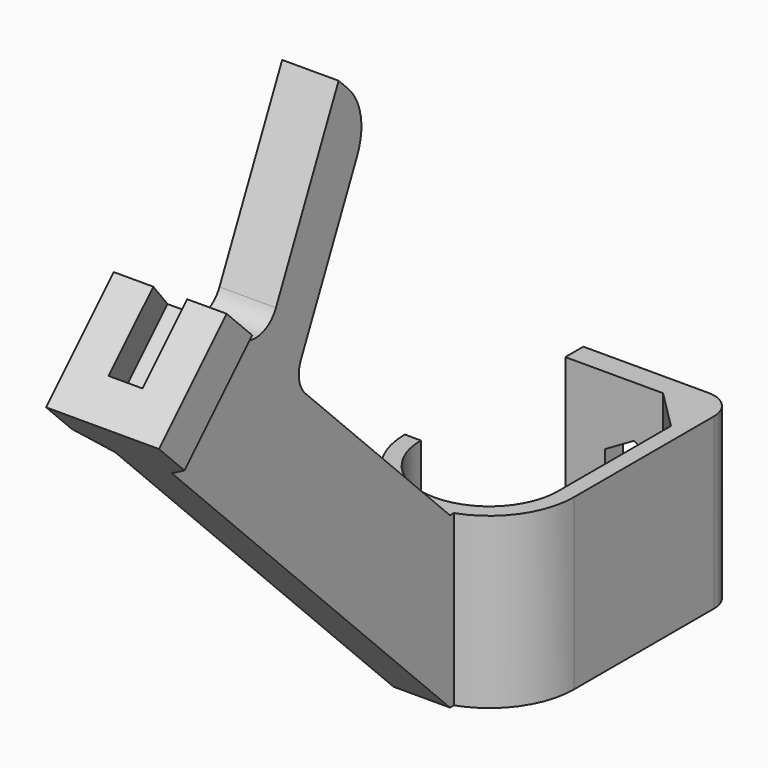
from build123d import *

# Parameters (mm, degrees)
F1_DEPTH  = 38.1
F2_W      = 3.6068
F2_H      = 38.1
F3_DEPTH  = 6.35
F5_DEPTH  = 12.7
F6_R      = 6.35
F7_R      = 12.7
F8_W      = 6.35
F8_H      = 10.16
F9_DEPTH  = 26.9407683632
F11_DEPTH = 17.78
F13_DEPTH = 25.4


# Not quite as in the source:
# - a feature names something its author has since deleted; it is built from what else it names


with BuildPart() as f1:
    # F0 (on Top) → F1 (new body)
    with BuildSketch(Plane.XY):
        with BuildLine():
            ThreePointArc((15.4432, 0), (0, -15.4432), (-15.4432, 0))
            Line((-15.4432, 0), (-19.05, 0))
            ThreePointArc((-19.05, 0), (0, -19.05), (19.05, 0))
            Line((19.05, 0), (19.05, 39.37))
            ThreePointArc((19.05, 39.37), (17.1901280605, 43.8601280605), (12.7, 45.72))
            Line((12.7, 45.72), (-15.4432, 45.72))
            Line((-15.4432, 45.72), (-15.4432, 40.64))
            Line((-15.4432, 40.64), (6.5532, 40.64))
            Line((6.5532, 40.64), (9.0932, 40.64))
            Line((9.0932, 40.64), (15.4432, 40.64))
            Line((15.4432, 40.64), (15.4432, 34.29))
            Line((15.4432, 34.29), (15.4432, 31.75))
            Line((15.4432, 31.75), (15.4432, 0))
        make_face()
        with BuildLine():
            Line((6.5532, 40.64), (15.4432, 31.75))
            Line((15.4432, 31.75), (15.4432, 34.29))
            ThreePointArc((15.4432, 34.29), (13.5833280605, 38.7801280605), (9.0932, 40.64))
            Line((9.0932, 40.64), (6.5532, 40.64))
        make_face()
        with BuildLine():
            ThreePointArc((9.0932, 40.64), (13.5833280605, 38.7801280605), (15.4432, 34.29))
            Line((15.4432, 34.29), (15.4432, 40.64))
            Line((15.4432, 40.64), (9.0932, 40.64))
        make_face()
    extrude(amount=F1_DEPTH)

    # F2 (on Right) → F3 (join, symmetric)
    with BuildSketch(Plane.YZ):
        Polygon((-108.8525612107, 89.8025612107), (-19.05, 0), (-19.05, 38.1), (-89.8025612107, 108.8525612107), align=None)
        with Locations((-17.2466, 19.05)):
            Rectangle(F2_W, F2_H)
    extrude(amount=F3_DEPTH, both=True)

    # F4 (on face) → F5 (join, through all)
    with BuildSketch(Plane.YZ.offset(6.35)):
        Polygon((-50.3730412721, 136.93248455), (-71.8420489686, 90.8920489686), (-62.8617928475, 81.9117928475), (-41.3927851511, 127.9522284289), align=None)
    extrude(amount=-F5_DEPTH)

    # F6
    f6_edges = [f1.edges().sort_by_distance(p)[0] for p in [
        (0, -71.842049, 90.892049),
        (0, -62.861793, 81.911793),
    ]]
    fillet(f6_edges, radius=F6_R)

    # F7
    f7_edges = [f1.edges().sort_by_distance(p)[0] for p in [
        (0, -41.392785, 127.952228),
    ]]
    fillet(f7_edges, radius=F7_R)

    # F8 (on face) → F9 (join, through all)
    with BuildSketch(Plane(origin=(0, 9.525, 9.525), x_dir=(1, 0, 0), z_dir=(0, 0.7071067812, 0.7071067812))):
        with Locations((-9.525, -135.3903841816)):
            Rectangle(F8_W, F8_H)
        with Locations((9.525, -135.3903841816)):
            Rectangle(F8_W, F8_H)
        Polygon((-12.7, -130.3103841816), (-6.35, -130.3103841816), (-6.35, -124.1391240244), align=None)
        Polygon((6.35, -124.1391240244), (6.35, -130.3103841816), (12.7, -130.3103841816), align=None)
    extrude(amount=-F9_DEPTH)

    # F10 (on face) → F11 (cut)
    with BuildSketch(Plane(origin=(0, 9.525, 9.525), x_dir=(1, 0, 0), z_dir=(0, 0.7071067812, 0.7071067812))):
        Polygon((-6.35, -130.3103841816), (-3.81, -140.4703841816), (0, -140.4703841816), (0, -130.3103841816), align=None)
        Polygon((0, -130.3103841816), (0, -140.4703841816), (3.81, -140.4703841816), (6.35, -130.3103841816), align=None)
    extrude(amount=-F11_DEPTH, mode=Mode.SUBTRACT)

    # F12 (on face) → F13 (cut)
    with BuildSketch(Plane(origin=(0, 45.72, 0), x_dir=(-1, 0, 0), z_dir=(0, 1, 0))):
        with BuildLine():
            Line((-6.477, 15.3105023065), (-3.2384999613, 13.4407534373))
            ThreePointArc((-3.2384999613, 13.4407534373), (-5.6092465291, 15.8114999806), (-6.477, 19.05))
            Line((-6.477, 19.05), (-6.477, 15.3105023065))
        make_face()
        with BuildLine():
            Line((-3.2384999613, 13.4407534373), (0, 11.5710046129))
            Line((0, 11.5710046129), (0, 12.573))
            ThreePointArc((0, 12.573), (-1.6763709335, 12.7936984173), (-3.2384999613, 13.4407534373))
        make_face()
        with BuildLine():
            Line((0, 12.573), (0, 11.5710046129))
            Line((0, 11.5710046129), (3.2384995854, 13.4407532203))
            ThreePointArc((3.2384995854, 13.4407532203), (1.6763707239, 12.7936983612), (0, 12.573))
        make_face()
        with BuildLine():
            ThreePointArc((6.477, 19.05), (5.6092464206, 15.8114997927), (3.2384995854, 13.4407532203))
            Line((3.2384995854, 13.4407532203), (6.477, 15.3105023065))
            Line((6.477, 15.3105023065), (6.477, 19.05))
        make_face()
        with BuildLine():
            ThreePointArc((3.2384999681, 24.6592465587), (5.6092465311, 22.288500016), (6.477, 19.05))
            Line((6.477, 19.05), (6.477, 22.7894976935))
            Line((6.477, 22.7894976935), (3.2384999681, 24.6592465587))
        make_face()
        with BuildLine():
            Line((-6.477, 22.7894976935), (-6.477, 19.05))
            ThreePointArc((-6.477, 19.05), (-5.6092466761, 22.2884997648), (-3.2385004704, 24.6592462687))
            Line((-3.2385004704, 24.6592462687), (-6.477, 22.7894976935))
        make_face()
        with BuildLine():
            ThreePointArc((-3.2385004704, 24.6592462687), (-1.6763712174, 25.3063015066), (0, 25.527))
            Line((0, 25.527), (0, 26.5289953871))
            Line((0, 26.5289953871), (-3.2385004704, 24.6592462687))
        make_face()
        with BuildLine():
            ThreePointArc((0, 25.527), (1.6763709373, 25.3063015816), (3.2384999681, 24.6592465587))
            Line((3.2384999681, 24.6592465587), (0, 26.5289953871))
            Line((0, 26.5289953871), (0, 25.527))
        make_face()
        with BuildLine():
            Line((0, 19.05), (6.477, 19.05))
            ThreePointArc((6.477, 19.05), (5.6092465311, 22.288500016), (3.2384999681, 24.6592465587))
            ThreePointArc((3.2384999681, 24.6592465587), (1.6763709373, 25.3063015816), (0, 25.527))
            Line((0, 25.527), (0, 19.05))
        make_face()
        with BuildLine():
            Line((-6.477, 19.05), (0, 19.05))
            Line((0, 19.05), (0, 25.527))
            ThreePointArc((0, 25.527), (-1.6763712174, 25.3063015066), (-3.2385004704, 24.6592462687))
            ThreePointArc((-3.2385004704, 24.6592462687), (-5.6092466761, 22.2884997648), (-6.477, 19.05))
        make_face()
        with BuildLine():
            ThreePointArc((-3.2384999613, 13.4407534373), (-1.6763709335, 12.7936984173), (0, 12.573))
            Line((0, 12.573), (0, 19.05))
            Line((0, 19.05), (-6.477, 19.05))
            ThreePointArc((-6.477, 19.05), (-5.6092465291, 15.8114999806), (-3.2384999613, 13.4407534373))
        make_face()
        with BuildLine():
            Line((0, 19.05), (0, 12.573))
            ThreePointArc((0, 12.573), (1.6763707239, 12.7936983612), (3.2384995854, 13.4407532203))
            ThreePointArc((3.2384995854, 13.4407532203), (5.6092464206, 15.8114997927), (6.477, 19.05))
            Line((6.477, 19.05), (0, 19.05))
        make_face()
    extrude(amount=-F13_DEPTH, mode=Mode.SUBTRACT)


solid = f1.part
